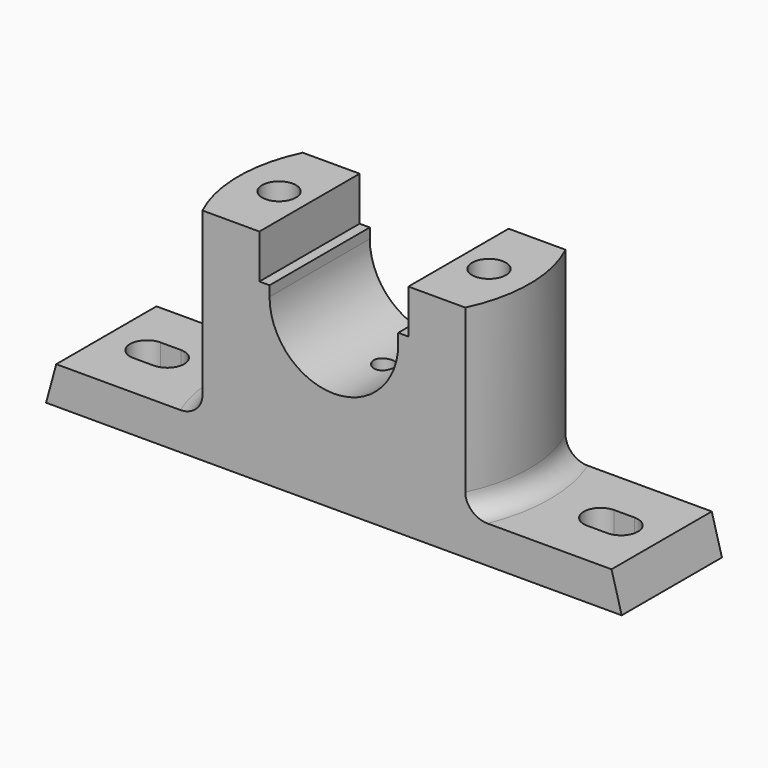
from build123d import *

# Parameters (mm, degrees)
F1_DEPTH  = 18.5
F3_DEPTH  = 54
F5_DEPTH  = 48.5
F6_R      = 5
F7_DEPTH  = 65.001
F8_W      = 20
F8_H      = 20
F9_DEPTH  = 8
F10_W     = 71
F10_H     = 2
F11_DEPTH = 11
F13_DEPTH = 11.001
F17_R     = 6


# Not quite as in the source:
# - a pattern or mirror of a feature is missing from the dataset's text; its kind, count and spacing are read off the source's solid


with BuildPart() as f1:
    # F0 (on Front) → F1 (new body, symmetric)
    with BuildSketch(Plane.XZ):
        Polygon((-82, 11), (-85, 0), (85, 0), (82, 11), align=None)
    extrude(amount=F1_DEPTH, both=True)

    # F2 (on face) → F3 (join)
    with BuildSketch(Plane.XY.offset(11)):
        with BuildLine():
            Line((38.8168777724, 18.5), (-38.8168777724, 18.5))
            ThreePointArc((-38.8168777724, 18.5), (-43, 0), (-38.8168777724, -18.5))
            Line((-38.8168777724, -18.5), (38.8168777724, -18.5))
            ThreePointArc((38.8168777724, -18.5), (43, 0), (38.8168777724, 18.5))
        make_face()
    extrude(amount=F3_DEPTH)

    # F4 (on Front) → F5 (cut, symmetric)
    with BuildSketch(Plane.XZ):
        with BuildLine():
            Line((22, 65), (-22, 65))
            Line((-22, 65), (-22, 52))
            Line((-22, 52), (-19, 52))
            Line((-19, 52), (-19, 49))
            ThreePointArc((-19, 49), (0, 30), (19, 49))
            Line((19, 49), (19, 52))
            Line((19, 52), (22, 52))
            Line((22, 52), (22, 65))
        make_face()
    extrude(amount=F5_DEPTH, both=True, mode=Mode.SUBTRACT)

    # F6 (on face) → F7 (cut, through all)
    with BuildSketch(Plane.XY.offset(65)):
        with Locations((-31, 0)):
            Circle(F6_R)
        with Locations((31, 0)):
            Circle(F6_R)
    extrude(amount=-F7_DEPTH, mode=Mode.SUBTRACT)

    # F8 (on face) → F9 (cut)
    with BuildSketch(Plane(origin=(0, 0, 0), x_dir=(1, 0, 0), z_dir=(0, 0, -1))):
        with Locations((-31, 0)):
            Rectangle(F8_W, F8_H)
        with Locations((31, 0)):
            Rectangle(F8_W, F8_H)
    extrude(amount=-F9_DEPTH, mode=Mode.SUBTRACT)

    # F10 (on Front) → F11 (cut, symmetric)
    with BuildSketch(Plane.XZ):
        with Locations((-39.5, 1)):
            Rectangle(F10_W, F10_H)
    f11 = extrude(amount=F11_DEPTH, both=True, mode=Mode.SUBTRACT)

    # F11_copies: F11 across plane
    add(f11.mirror(Plane(origin=(0, 0, 0), x_dir=(0, 0, 1), z_dir=(1, 0, 0))), mode=Mode.SUBTRACT)

    # F12 (on face) → F13 (cut, through all)
    with BuildSketch(Plane.XY.offset(11)):
        with BuildLine():
            ThreePointArc((-70, 5), (-75, 0), (-70, -5))
            Line((-70, -5), (-64, -5))
            ThreePointArc((-64, -5), (-59, 0), (-64, 5))
            Line((-64, 5), (-70, 5))
        make_face()
        with BuildLine():
            ThreePointArc((70, -5), (75, 0), (70, 5))
            Line((70, 5), (64, 5))
            ThreePointArc((64, 5), (59, 0), (64, -5))
            Line((64, -5), (70, -5))
        make_face()
    extrude(amount=-F13_DEPTH, mode=Mode.SUBTRACT)

    # F14 (on Front) → F15 (revolve, cut)
    with BuildSketch(Plane.XZ):
        Polygon((3, 31.8085759505), (0, 31.8085759505), (0, 22.1974181429), (3, 24), align=None)
    revolve(axis=Axis((0, 0, 27.0029970467), (0, 0, -1)), mode=Mode.SUBTRACT)

    # F14 (on Front) → F16 (revolve, cut)
    with BuildSketch(Plane.XZ):
        Polygon((3, 31.8085759505), (0, 31.8085759505), (0, 22.1974181429), (3, 24), align=None)
    revolve(axis=Axis((0, 0, 27.0029970467), (0, 0, -1)), mode=Mode.SUBTRACT)

    # F17
    f17_edges = [f1.edges().sort_by_distance(p)[0] for p in [
        (43, 0, 11),
        (-43, 0, 11),
    ]]
    fillet(f17_edges, radius=F17_R)


solid = f1.part
